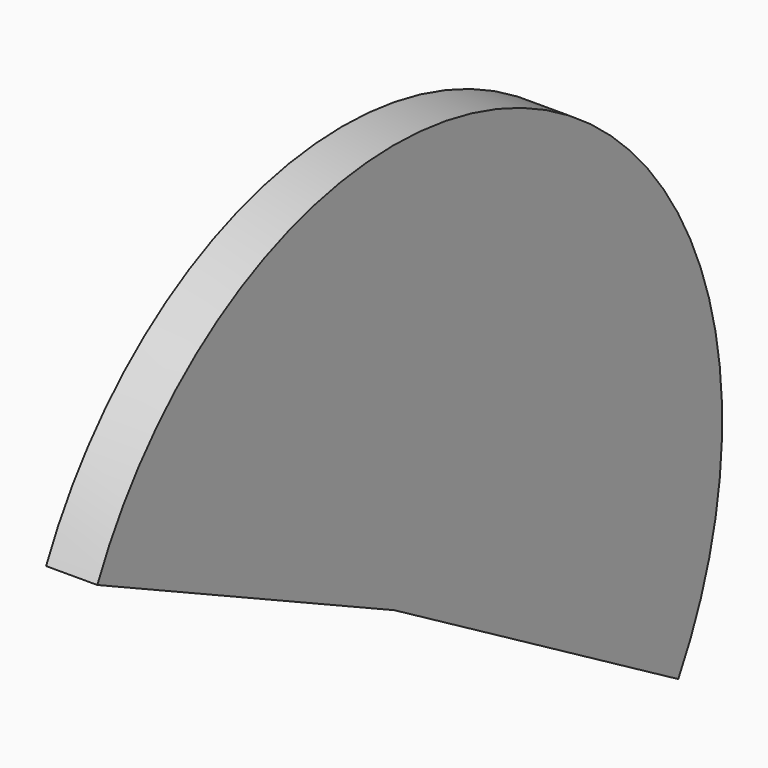
from build123d import *

# Parameters (mm, degrees)
F1_ANGLE_BACK = 65
F1_ANGLE      = 185


# Not quite as in the source:
# - a feature of the source that left no trace in its solid (it failed there, or was rolled back) is left out


with BuildPart() as f1:
    # F0 (on Front) → F1 (revolve)
    with BuildSketch(Plane.XZ, mode=Mode.PRIVATE) as f1_sk:
        with BuildLine():
            Line((-15.24, 0), (0, 0))
            Line((0, 0), (0, 50.8))
            Line((0, 50.8), (-6.35, 50.8))
            Line((-6.35, 50.8), (-4.7617064118, 41.792339449))
            ThreePointArc((-4.7617064118, 41.792339449), (-4.8311637627, 41.5331210865), (-5.0743828734, 41.4197061526))
            Line((-5.0743828734, 41.4197061526), (-6.2835011077, 41.4197061526))
            ThreePointArc((-6.2835011077, 41.4197061526), (-6.5080075107, 41.3267125556), (-6.6010011077, 41.1022061526))
            Line((-6.6010011077, 41.1022061526), (-6.6010011077, 40.4672061526))
            ThreePointArc((-6.6010011077, 40.4672061526), (-6.5080075107, 40.2426997495), (-6.2835011077, 40.1497061526))
            Line((-6.2835011077, 40.1497061526), (-5.0743828734, 40.1497061526))
            ThreePointArc((-5.0743828734, 40.1497061526), (-4.8311637627, 40.0362912186), (-4.7617064118, 39.7770728561))
            Line((-4.7617064118, 39.7770728561), (-5.2010717431, 37.2853082403))
            ThreePointArc((-5.2010717431, 37.2853082403), (-5.3096631386, 37.0972224261), (-5.5137482047, 37.0229415367))
            Line((-5.5137482047, 37.0229415367), (-6.8348340718, 37.0229415367))
            ThreePointArc((-6.8348340718, 37.0229415367), (-7.0593404748, 36.9299479398), (-7.1523340718, 36.7054415367))
            Line((-7.1523340718, 36.7054415367), (-7.1523340718, 36.0704415367))
            ThreePointArc((-7.1523340718, 36.0704415367), (-7.2453276688, 35.8459351337), (-7.4698340718, 35.7529415367))
            Line((-7.4698340718, 35.7529415367), (-8.7398340718, 35.7529415367))
            ThreePointArc((-8.7398340718, 35.7529415367), (-8.9643404748, 35.6599479398), (-9.0573340718, 35.4354415367))
            Line((-9.0573340718, 35.4354415367), (-9.0573340718, 34.8004415367))
            ThreePointArc((-9.0573340718, 34.8004415367), (-8.9643404748, 34.5759351337), (-8.7398340718, 34.4829415367))
            Line((-8.7398340718, 34.4829415367), (-3.5686493249, 34.4829415367))
            ThreePointArc((-3.5686493249, 34.4829415367), (-3.3254302142, 34.3695266028), (-3.2559728633, 34.1103082403))
            Line((-3.2559728633, 34.1103082403), (-7.113602572, 12.2326030065))
            ThreePointArc((-7.113602572, 12.2326030065), (-7.2221939675, 12.0445171922), (-7.4262790336, 11.9702363029))
            Line((-7.4262790336, 11.9702363029), (-8.1123649007, 11.9702363029))
            ThreePointArc((-8.1123649007, 11.9702363029), (-8.3368713037, 11.8772427059), (-8.4298649007, 11.6527363029))
            Line((-8.4298649007, 11.6527363029), (-8.4298649007, 8.9432889844))
            ThreePointArc((-8.4298649007, 8.9432889844), (-8.4596121783, 8.8091076862), (-8.5432798346, 8.7000698737))
            Line((-8.5432798346, 8.7000698737), (-15.1265850661, 3.176020882))
            ThreePointArc((-15.1265850661, 3.176020882), (-15.2102527224, 3.0669830694), (-15.24, 2.9328017713))
            Line((-15.24, 2.9328017713), (-15.24, 0))
        make_face()
    revolve(f1_sk.sketch.rotate(Axis((-7.62, 0, 0), (-1, 0, 0)), -F1_ANGLE_BACK), axis=Axis((-7.62, 0, 0), (-1, 0, 0)), revolution_arc=F1_ANGLE)


solid = f1.part
